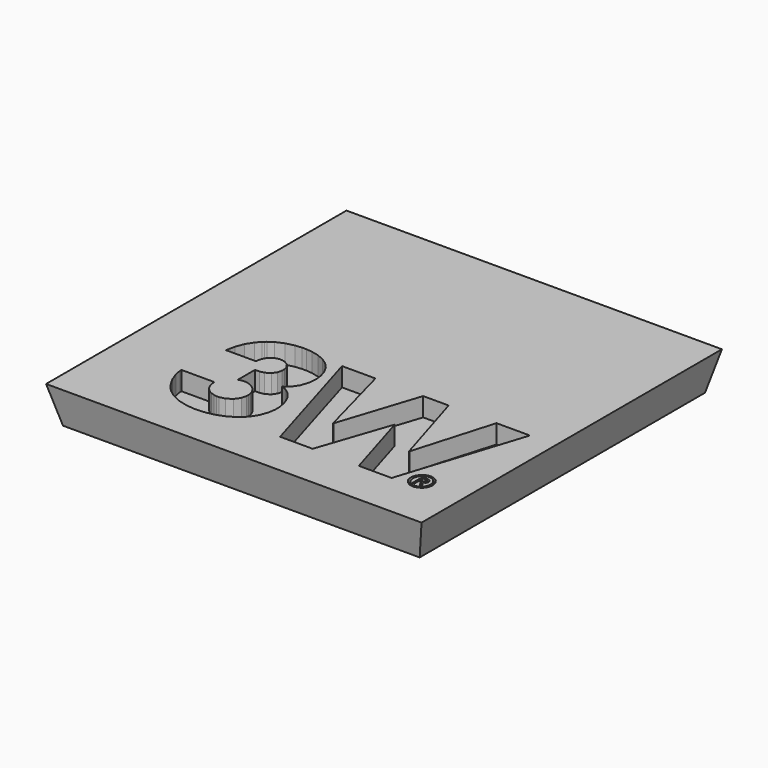
from build123d import *

# Parameters (mm, degrees)
F0_W     = 199.988932
F0_H     = 199.988932
F1_DEPTH = 20
F2_DEPTH = 10
F3_DEPTH = 18
F4_SIZE2 = 19.99999
F4_SIZE  = 4.99999


# Not quite as in the source:
# - a fillet or chamfer is up to 0.001 mm smaller than in the source, because OpenCascade refuses the exact size


with BuildPart() as f1:
    # F0 (on Top) → F1 (new body)
    with BuildSketch(Plane.XY):
        Rectangle(F0_W, F0_H)
        Polygon((-44.50207, -29.509212), (-60.447428, -29.509212), (-60.322206, -28.28417), (-59.539378, -24.651716), (-57.91327, -20.393406), (-55.631334, -16.723614), (-53.542184, -14.331442), (-52.75834, -13.634212), (-51.972464, -12.934188), (-49.317148, -11.168888), (-45.331888, -9.392666), (-40.87241, -8.316214), (-37.219382, -7.955534), (-36.001198, -7.955534), (-34.930334, -7.955534), (-31.715456, -8.270748), (-27.745182, -9.210548), (-24.17064, -10.75817), (-21.070062, -12.89685), (-18.522188, -15.614142), (-16.603726, -18.89252), (-15.395194, -22.718268), (-14.975078, -25.98547), (-14.975078, -27.075638), (-14.975078, -28.059634), (-15.376144, -31.011114), (-16.616172, -34.78276), (-18.756376, -38.077648), (-20.99691, -40.107616), (-21.85416, -40.587422), (-21.218906, -40.753792), (-19.38909, -41.549066), (-17.232122, -43.002962), (-15.392654, -44.861988), (-13.873988, -47.038006), (-12.681966, -49.443894), (-11.824716, -51.992022), (-11.30554, -54.595268), (-11.130534, -56.524144), (-11.130534, -57.168034), (-11.130534, -58.43397), (-11.692382, -62.23635), (-13.286994, -66.64452), (-15.772892, -70.390004), (-19.011138, -73.46442), (-22.862794, -75.8650248), (-27.189938, -77.5848334), (-31.850584, -78.6211026), (-35.49269, -78.968346), (-36.70681, -78.968346), (-38.079172, -78.968346), (-42.196766, -78.5687278), (-47.346616, -77.2871454), (-52.08016, -74.9940842), (-55.372254, -72.527414), (-56.320182, -71.559928), (-57.10301, -70.756526), (-59.171332, -68.080382), (-61.613288, -63.917322), (-63.286132, -59.430666), (-63.869316, -56.085994), (-63.834772, -54.979316), (-46.372272, -54.979316), (-46.372272, -55.453534), (-46.201584, -56.879744), (-45.703744, -58.64225), (-44.90339, -60.23102), (-43.824144, -61.610494), (-42.49039, -62.746128), (-40.926004, -63.600584), (-39.1541, -64.139064), (-37.689282, -64.32804), (-37.200078, -64.32804), (-36.292028, -64.32804), (-33.564576, -63.69812), (-30.657038, -61.915294), (-28.727654, -59.132978), (-28.027884, -56.414162), (-28.027884, -55.508398), (-28.027884, -55.056532), (-28.22067, -53.700426), (-28.770326, -52.0319), (-29.631894, -50.532538), (-30.76321, -49.23282), (-32.117792, -48.167798), (-33.654238, -47.36719), (-35.327082, -46.863), (-36.652962, -46.68901), (-37.093906, -46.68901), (-37.474144, -46.68901), (-38.615366, -46.84776), (-39.819834, -47.147988), (-40.05834, -47.218092), (-40.05834, -35.788854), (-38.3286, -35.788854), (-37.574728, -35.788854), (-35.309556, -35.292792), (-32.932116, -33.865312), (-31.373572, -31.591504), (-30.81401, -29.314648), (-30.81401, -28.556966), (-30.81401, -27.873198), (-31.32709, -25.82291), (-32.73806, -23.73249), (-34.86277, -22.394418), (-36.854384, -21.924518), (-37.516816, -21.924518), (-38.254178, -21.924518), (-40.46474, -22.508464), (-42.677588, -24.115522), (-44.055792, -26.522934), (-44.514516, -28.763722), align=None, mode=Mode.SUBTRACT)
        Polygon((77.440536, -76.8172454), (76.887578, -76.8172454), (76.303378, -76.8172454), (74.554588, -76.3679956), (72.724772, -75.1277644), (71.529956, -73.259188), (71.102728, -71.509128), (71.102728, -70.926198), (71.102728, -70.32244), (71.569834, -68.515992), (72.83069, -66.656966), (74.67473, -65.458086), (76.333858, -65.033652), (76.887578, -65.033652), (77.439012, -65.033652), (79.095346, -65.458086), (80.92694, -66.656966), (82.17535, -68.515992), (82.638138, -70.32244), (82.638138, -70.926198), (82.64398, -71.525638), (82.19059, -73.33361), (80.940656, -75.193906), (79.100934, -76.3928114), align=None, mode=Mode.SUBTRACT)
        Polygon((3.898646, -10.565384), (15.327884, -53.03901), (15.50416, -53.03901), (29.298646, -10.565384), (42.880534, -10.565384), (55.792878, -53.03901), (55.969408, -53.03901), (68.350638, -10.565384), (86.165944, -10.565384), (65.141602, -76.3583436), (47.679102, -76.3583436), (36.177728, -38.222428), (36.001452, -38.222428), (23.089108, -76.3583436), (5.73278, -76.3583436), (-13.91666, -10.565384), align=None, mode=Mode.SUBTRACT)
    extrude(amount=F1_DEPTH)

    # F0 (on Top) → F2 (join)
    with BuildSketch(Plane.XY):
        Polygon((15.50416, -53.03901), (15.327884, -53.03901), (3.898646, -10.565384), (-13.91666, -10.565384), (5.73278, -76.3583436), (23.089108, -76.3583436), (36.001452, -38.222428), (36.177728, -38.222428), (47.679102, -76.3583436), (65.141602, -76.3583436), (86.165944, -10.565384), (68.350638, -10.565384), (55.969408, -53.03901), (55.792878, -53.03901), (42.880534, -10.565384), (29.298646, -10.565384), align=None)
        Polygon((-60.322206, -28.28417), (-60.447428, -29.509212), (-44.50207, -29.509212), (-44.514516, -28.763722), (-44.055792, -26.522934), (-42.677588, -24.115522), (-40.46474, -22.508464), (-38.254178, -21.924518), (-37.516816, -21.924518), (-36.854384, -21.924518), (-34.86277, -22.394418), (-32.73806, -23.73249), (-31.32709, -25.82291), (-30.81401, -27.873198), (-30.81401, -28.556966), (-30.81401, -29.314648), (-31.373572, -31.591504), (-32.932116, -33.865312), (-35.309556, -35.292792), (-37.574728, -35.788854), (-38.3286, -35.788854), (-40.05834, -35.788854), (-40.05834, -47.218092), (-39.819834, -47.147988), (-38.615366, -46.84776), (-37.474144, -46.68901), (-37.093906, -46.68901), (-36.652962, -46.68901), (-35.327082, -46.863), (-33.654238, -47.36719), (-32.117792, -48.167798), (-30.76321, -49.23282), (-29.631894, -50.532538), (-28.770326, -52.0319), (-28.22067, -53.700426), (-28.027884, -55.056532), (-28.027884, -55.508398), (-28.027884, -56.414162), (-28.727654, -59.132978), (-30.657038, -61.915294), (-33.564576, -63.69812), (-36.292028, -64.32804), (-37.200078, -64.32804), (-37.689282, -64.32804), (-39.1541, -64.139064), (-40.926004, -63.600584), (-42.49039, -62.746128), (-43.824144, -61.610494), (-44.90339, -60.23102), (-45.703744, -58.64225), (-46.201584, -56.879744), (-46.372272, -55.453534), (-46.372272, -54.979316), (-63.834772, -54.979316), (-63.869316, -56.085994), (-63.286132, -59.430666), (-61.613288, -63.917322), (-59.171332, -68.080382), (-57.10301, -70.756526), (-56.320182, -71.559928), (-55.372254, -72.527414), (-52.08016, -74.9940842), (-47.346616, -77.2871454), (-42.196766, -78.5687278), (-38.079172, -78.968346), (-36.70681, -78.968346), (-35.49269, -78.968346), (-31.850584, -78.6211026), (-27.189938, -77.5848334), (-22.862794, -75.8650248), (-19.011138, -73.46442), (-15.772892, -70.390004), (-13.286994, -66.64452), (-11.692382, -62.23635), (-11.130534, -58.43397), (-11.130534, -57.168034), (-11.130534, -56.524144), (-11.30554, -54.595268), (-11.824716, -51.992022), (-12.681966, -49.443894), (-13.873988, -47.038006), (-15.392654, -44.861988), (-17.232122, -43.002962), (-19.38909, -41.549066), (-21.218906, -40.753792), (-21.85416, -40.587422), (-20.99691, -40.107616), (-18.756376, -38.077648), (-16.616172, -34.78276), (-15.376144, -31.011114), (-14.975078, -28.059634), (-14.975078, -27.075638), (-14.975078, -25.98547), (-15.395194, -22.718268), (-16.603726, -18.89252), (-18.522188, -15.614142), (-21.070062, -12.89685), (-24.17064, -10.75817), (-27.745182, -9.210548), (-31.715456, -8.270748), (-34.930334, -7.955534), (-36.001198, -7.955534), (-37.219382, -7.955534), (-40.87241, -8.316214), (-45.331888, -9.392666), (-49.317148, -11.168888), (-51.972464, -12.934188), (-52.75834, -13.634212), (-53.542184, -14.331442), (-55.631334, -16.723614), (-57.91327, -20.393406), (-59.539378, -24.651716), align=None)
    extrude(amount=F2_DEPTH)



with BuildPart() as f1b:
    # F0 (on Top) → F1, piece 2 (new body)
    with BuildSketch(Plane.XY):
        Polygon((77.117956, -66.057526), (76.887578, -66.057526), (76.656184, -66.057526), (75.961494, -66.148458), (75.104752, -66.41592), (74.331322, -66.844418), (73.658984, -67.418966), (73.106534, -68.128642), (72.690228, -68.95973), (72.428608, -69.895466), (72.337422, -70.668388), (72.337422, -70.926198), (72.337422, -71.170038), (72.416162, -71.904606), (72.65035, -72.81672), (73.032112, -73.643744), (73.554336, -74.364342), (74.207624, -74.9596672), (74.986134, -75.4088916), (75.881738, -75.6941336), (76.63561, -75.793346), (76.887578, -75.793346), (77.115162, -75.793346), (77.799946, -75.7023886), (78.650338, -75.4391938), (79.416402, -75.0147598), (80.08493, -74.444352), (80.63484, -73.735946), (81.049368, -72.906382), (81.311496, -71.965058), (81.403444, -71.185278), (81.403444, -70.926198), (81.403444, -70.665594), (81.312512, -69.885814), (81.054956, -68.94449), (80.644238, -68.113656), (80.098646, -67.40652), (79.432912, -66.834766), (78.664308, -66.410332), (77.811122, -66.147188), align=None)
        Polygon((75.724766, -71.45528), (75.724766, -74.277474), (74.666602, -74.277474), (74.666602, -67.751198), (77.13599, -67.751198), (77.394816, -67.751198), (78.17358, -67.85864), (78.912212, -68.194936), (79.353156, -68.776342), (79.499206, -69.408802), (79.499206, -69.619622), (79.499206, -69.807074), (79.368396, -70.3707), (79.008478, -70.898512), (78.471268, -71.226426), (77.973682, -71.364348), (77.805534, -71.383652), (79.639668, -74.24166), (78.440788, -74.24166), (76.747116, -71.45528), align=None, mode=Mode.SUBTRACT)
    extrude(amount=F1_DEPTH)


with BuildPart() as f1c:
    # F0 (on Top) → F1, piece 3 (new body)
    with BuildSketch(Plane.XY):
        Polygon((75.724766, -70.573392), (76.923646, -70.573392), (77.068172, -70.573392), (77.502512, -70.54723), (77.986128, -70.41769), (78.316836, -70.11035), (78.440788, -69.68871), (78.440788, -69.549518), (78.440788, -69.432424), (78.308708, -69.083682), (77.972412, -68.816474), (77.517752, -68.695062), (77.15123, -68.66763), (77.029818, -68.66763), (75.724766, -68.66763), align=None)
    extrude(amount=F1_DEPTH)


with BuildPart() as f1_1:
    add(f1.part)

    add(f1b.part)  # F3 merges F1b

    add(f1c.part)  # F3 merges F1c
    # F0 (on Top) → F3 (join)
    with BuildSketch(Plane.XY):
        Polygon((76.303378, -76.8172454), (76.887578, -76.8172454), (77.440536, -76.8172454), (79.100934, -76.3928114), (80.940656, -75.193906), (82.19059, -73.33361), (82.64398, -71.525638), (82.638138, -70.926198), (82.638138, -70.32244), (82.17535, -68.515992), (80.92694, -66.656966), (79.095346, -65.458086), (77.439012, -65.033652), (76.887578, -65.033652), (76.333858, -65.033652), (74.67473, -65.458086), (72.83069, -66.656966), (71.569834, -68.515992), (71.102728, -70.32244), (71.102728, -70.926198), (71.102728, -71.509128), (71.529956, -73.259188), (72.724772, -75.1277644), (74.554588, -76.3679956), align=None)
        Polygon((76.656184, -66.057526), (76.887578, -66.057526), (77.117956, -66.057526), (77.811122, -66.147188), (78.664308, -66.410332), (79.432912, -66.834766), (80.098646, -67.40652), (80.644238, -68.113656), (81.054956, -68.94449), (81.312512, -69.885814), (81.403444, -70.665594), (81.403444, -70.926198), (81.403444, -71.185278), (81.311496, -71.965058), (81.049368, -72.906382), (80.63484, -73.735946), (80.08493, -74.444352), (79.416402, -75.0147598), (78.650338, -75.4391938), (77.799946, -75.7023886), (77.115162, -75.793346), (76.887578, -75.793346), (76.63561, -75.793346), (75.881738, -75.6941336), (74.986134, -75.4088916), (74.207624, -74.9596672), (73.554336, -74.364342), (73.032112, -73.643744), (72.65035, -72.81672), (72.416162, -71.904606), (72.337422, -71.170038), (72.337422, -70.926198), (72.337422, -70.668388), (72.428608, -69.895466), (72.690228, -68.95973), (73.106534, -68.128642), (73.658984, -67.418966), (74.331322, -66.844418), (75.104752, -66.41592), (75.961494, -66.148458), align=None, mode=Mode.SUBTRACT)
        Polygon((74.666602, -74.277474), (75.724766, -74.277474), (75.724766, -71.45528), (76.747116, -71.45528), (78.440788, -74.24166), (79.639668, -74.24166), (77.805534, -71.383652), (77.973682, -71.364348), (78.471268, -71.226426), (79.008478, -70.898512), (79.368396, -70.3707), (79.499206, -69.807074), (79.499206, -69.619622), (79.499206, -69.408802), (79.353156, -68.776342), (78.912212, -68.194936), (78.17358, -67.85864), (77.394816, -67.751198), (77.13599, -67.751198), (74.666602, -67.751198), align=None)
        Polygon((77.068172, -70.573392), (76.923646, -70.573392), (75.724766, -70.573392), (75.724766, -68.66763), (77.029818, -68.66763), (77.15123, -68.66763), (77.517752, -68.695062), (77.972412, -68.816474), (78.308708, -69.083682), (78.440788, -69.432424), (78.440788, -69.549518), (78.440788, -69.68871), (78.316836, -70.11035), (77.986128, -70.41769), (77.502512, -70.54723), align=None, mode=Mode.SUBTRACT)
    extrude(amount=F3_DEPTH)

    # F4 (size 5 and 20 in the source; OpenCascade refuses exactly that, so slightly less here)
    f4_edges = [f1_1.edges().sort_by_distance(p)[0] for p in [
        (0, -99.994466, 0),
        (-99.994466, 0, 0),
        (99.994466, 0, 0),
        (0, 99.994466, 0),
    ]]
    f4_side = f1_1.faces().sort_by_distance((0, 0, 0))[0]
    chamfer(f4_edges, length=F4_SIZE, length2=F4_SIZE2, reference=f4_side)


solid = f1_1.part
